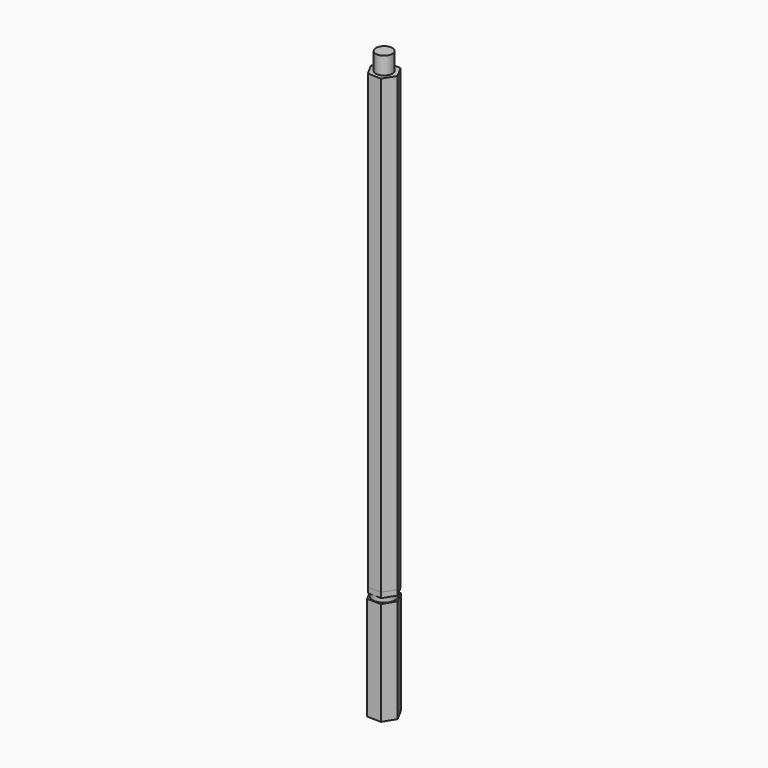
from build123d import *

# Parameters (mm, degrees)
F1_DEPTH = 133.35
F2_R     = 2.384296381
F3_DEPTH = 5.08
F4_DEPTH = 1.524
F5_R     = 3.2723319481
F6_DEPTH = 1.524
F8_DEPTH = 30.226


with BuildPart() as f1:
    # F0 (on Top) → F1 (new body)
    with BuildSketch(Plane.XY):
        Polygon((-41.5820354619, 36.8828393166), (-39.4786010631, 40.2483318945), (-41.3414859324, 43.7527058081), (-45.3078052006, 43.8915871437), (-47.4112395994, 40.5260945657), (-45.5483547301, 37.0217206522), align=None)
    extrude(amount=-F1_DEPTH)

    # F2 (on face) → F3 (join)
    with BuildSketch(Plane.XY):
        with Locations((-43.4742867947, 40.3853803873)):
            Circle(F2_R)
    extrude(amount=F3_DEPTH)


with BuildPart() as f4:
    # F4 (new): a face of the model
    f4_faces = [f1.part.faces().sort_by_distance(p)[0] for p in [
        (-43.4449203312, 40.3872132301, -133.35),
    ]]
    extrude(f4_faces, amount=-F4_DEPTH)


with BuildPart() as f6:
    # F5 (on face) → F6 (new body)
    with BuildSketch(Plane(origin=(0, 0, -133.35), x_dir=(1, 0, 0), z_dir=(0, 0, -1))):
        with Locations((-43.565195096, -40.4523536563)):
            Circle(F5_R)
    extrude(amount=F6_DEPTH)

    # F7 (on face) → F8 (join)
    with BuildSketch(Plane(origin=(0, 0, -134.874), x_dir=(1, 0, 0), z_dir=(0, 0, -1))):
        Polygon((-39.4883785057, -40.355072412), (-41.6110348297, -36.8730863004), (-45.68785142, -36.9703675446), (-47.6420116863, -40.5496349006), (-45.5193553623, -44.0316210122), (-41.442538772, -43.9343397679), align=None)
    extrude(amount=F8_DEPTH)


solid = Compound([f1.part, f4.part, f6.part])
